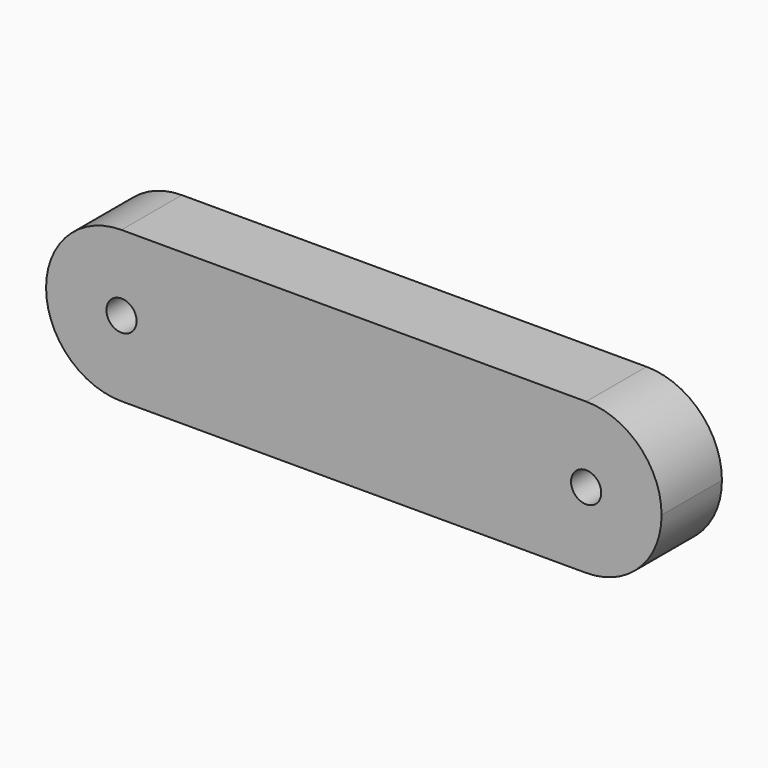
from build123d import *

# Parameters (mm, degrees)
F3_DEPTH = 5
F4_D     = 2
F5_D     = 2


# Not quite as in the source:
# - a feature names something its author has since deleted; it is built from what else it names


with BuildPart() as f3:
    # F2 (on Front) → F3 (new body)
    with BuildSketch(Plane.XZ):
        with BuildLine():
            ThreePointArc((12.9616053321, -5), (16.4971392381, -3.5355339059), (17.9616053321, 0))
            ThreePointArc((17.9616053321, 0), (16.4971392381, 3.5355339059), (12.9616053321, 5))
            ThreePointArc((12.9616053321, 5), (7.9616053321, 0), (12.9616053321, -5))
        make_face()
        with BuildLine():
            ThreePointArc((12.9616053321, -5), (7.9616053321, 0), (12.9616053321, 5))
            Line((12.9616053321, 5), (-17.8376678377, 5))
            ThreePointArc((-17.8376678377, 5), (-14.3021339318, 3.5355339059), (-12.8376678377, 0))
            ThreePointArc((-12.8376678377, 0), (-14.3021339318, -3.5355339059), (-17.8376678377, -5))
            Line((-17.8376678377, -5), (12.9616053321, -5))
        make_face()
        with BuildLine():
            ThreePointArc((-12.8376678377, 0), (-14.3021339318, 3.5355339059), (-17.8376678377, 5))
            ThreePointArc((-17.8376678377, 5), (-22.8376678377, 0), (-17.8376678377, -5))
            ThreePointArc((-17.8376678377, -5), (-14.3021339318, -3.5355339059), (-12.8376678377, 0))
        make_face()
    extrude(amount=F3_DEPTH)

    # F4 (through all)
    with Locations(Plane(origin=(0, 0, 0), x_dir=(1, 0, 0), z_dir=(0, 1, 0))):
        with Locations((12.9616053321, 0)):
            Hole(F4_D / 2)

    # F5 (through all)
    with Locations(Plane(origin=(0, 0, 0), x_dir=(1, 0, 0), z_dir=(0, 1, 0))):
        with Locations((-17.8376678377, 0)):
            Hole(F5_D / 2)


solid = f3.part
